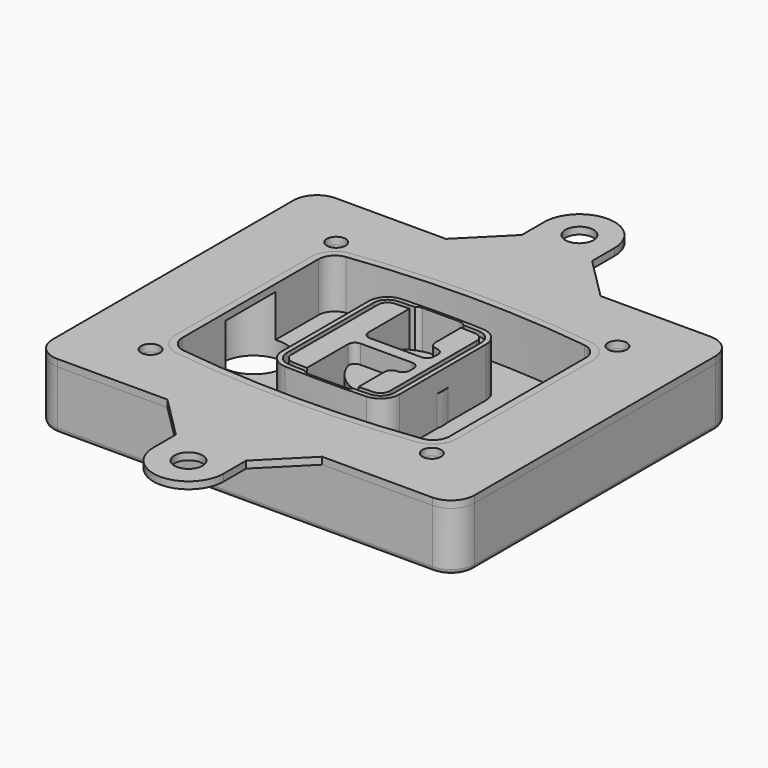
from build123d import *

# Parameters (mm, degrees)
F1_DEPTH  = 25
F2_DEPTH  = 3
F3_DEPTH  = 18
F5_DEPTH  = 21
F6_DEPTH  = 2
F8_DEPTH  = 20
F9_DEPTH  = 16
F10_DEPTH = 25
F7_R      = 6
F7_R_2    = 4
F11_DEPTH = 6
F13_DEPTH = 9
F15_R     = 2
F17_R     = 4
F17_R_2   = 6
F18_DEPTH = 3


# Not quite as in the source:
# - a feature of the source that left no trace in its solid (it failed there, or was rolled back) is left out
# - a feature names something its author has since deleted; it is built from what else it names


with BuildPart() as f1:
    # F0 (on Top) → F1 (new body)
    with BuildSketch(Plane.XY):
        with BuildLine():
            ThreePointArc((-90, -64.25), (-87.0710678119, -71.3210678119), (-80, -74.25))
            Line((-80, -74.25), (80, -74.25))
            ThreePointArc((80, -74.25), (87.0710678119, -71.3210678119), (90, -64.25))
            Line((90, -64.25), (90, 64.25))
            ThreePointArc((90, 64.25), (87.0710678119, 71.3210678119), (80, 74.25))
            Line((80, 74.25), (-80, 74.25))
            ThreePointArc((-80, 74.25), (-87.0710678119, 71.3210678119), (-90, 64.25))
            Line((-90, 64.25), (-90, -64.25))
        make_face()
        with BuildLine():
            ThreePointArc((-60.5228833457, 45.5343231338), (-62.6370880358, 52.5076181093), (-56, 49.5))
            ThreePointArc((-56, 49.5), (-56.010223193, 49.2142010667), (-56.0408405151, 48.9298630223))
            ThreePointArc((-56.0408405151, 48.9298630223), (-53.9627965672, 49.7276492937), (-51.7845761632, 50.1860000938))
            ThreePointArc((-51.7845761632, 50.1860000938), (0, 53.5), (51.7845761632, 50.1860000938))
            ThreePointArc((51.7845761632, 50.1860000938), (53.9627965672, 49.7276492937), (56.0408405151, 48.9298630223))
            ThreePointArc((56.0408405151, 48.9298630223), (59.7142010667, 53.489776807), (64, 49.5))
            ThreePointArc((64, 49.5), (63.0076181093, 46.8629119642), (60.5228833457, 45.5343231338))
            ThreePointArc((60.5228833457, 45.5343231338), (63.1019152577, 41.2337455934), (64, 36.300205629))
            Line((64, 36.300205629), (64, -36.300205629))
            ThreePointArc((64, -36.300205629), (63.1019152577, -41.2337455934), (60.5228833457, -45.5343231338))
            ThreePointArc((60.5228833457, -45.5343231338), (63.0076181093, -46.8629119642), (64, -49.5))
            ThreePointArc((64, -49.5), (59.7142010667, -53.489776807), (56.0408405151, -48.9298630223))
            ThreePointArc((56.0408405151, -48.9298630223), (53.9627965672, -49.7276492937), (51.7845761632, -50.1860000938))
            ThreePointArc((51.7845761632, -50.1860000938), (0, -53.5), (-51.7845761632, -50.1860000938))
            ThreePointArc((-51.7845761632, -50.1860000938), (-53.9627965672, -49.7276492937), (-56.0408405151, -48.9298630223))
            ThreePointArc((-56.0408405151, -48.9298630223), (-56.010223193, -49.2142010667), (-56, -49.5))
            ThreePointArc((-56, -49.5), (-62.6370880358, -52.5076181093), (-60.5228833457, -45.5343231338))
            ThreePointArc((-60.5228833457, -45.5343231338), (-63.1019152577, -41.2337455934), (-64, -36.300205629))
            Line((-64, -36.300205629), (-64, 36.300205629))
            ThreePointArc((-64, 36.300205629), (-63.1019152577, 41.2337455934), (-60.5228833457, 45.5343231338))
        make_face(mode=Mode.SUBTRACT)
        with BuildLine():
            ThreePointArc((-56.0408405151, 48.9298630223), (-57.584545341, 46.3116495189), (-60.5228833457, 45.5343231338))
            ThreePointArc((-60.5228833457, 45.5343231338), (-63.1019152577, 41.2337455934), (-64, 36.300205629))
            Line((-64, 36.300205629), (-64, -36.300205629))
            ThreePointArc((-64, -36.300205629), (-63.1019152577, -41.2337455934), (-60.5228833457, -45.5343231338))
            ThreePointArc((-60.5228833457, -45.5343231338), (-57.584545341, -46.3116495189), (-56.0408405151, -48.9298630223))
            ThreePointArc((-56.0408405151, -48.9298630223), (-53.9627965672, -49.7276492937), (-51.7845761632, -50.1860000938))
            ThreePointArc((-51.7845761632, -50.1860000938), (0, -53.5), (51.7845761632, -50.1860000938))
            ThreePointArc((51.7845761632, -50.1860000938), (53.9627965672, -49.7276492937), (56.0408405151, -48.9298630223))
            ThreePointArc((56.0408405151, -48.9298630223), (57.584545341, -46.3116495189), (60.5228833457, -45.5343231338))
            ThreePointArc((60.5228833457, -45.5343231338), (63.1019152577, -41.2337455934), (64, -36.300205629))
            Line((64, -36.300205629), (64, 36.300205629))
            ThreePointArc((64, 36.300205629), (63.1019152577, 41.2337455934), (60.5228833457, 45.5343231338))
            ThreePointArc((60.5228833457, 45.5343231338), (57.584545341, 46.3116495189), (56.0408405151, 48.9298630223))
            ThreePointArc((56.0408405151, 48.9298630223), (53.9627965672, 49.7276492937), (51.7845761632, 50.1860000938))
            ThreePointArc((51.7845761632, 50.1860000938), (0, 53.5), (-51.7845761632, 50.1860000938))
            ThreePointArc((-51.7845761632, 50.1860000938), (-53.9627965672, 49.7276492937), (-56.0408405151, 48.9298630223))
        make_face()
        with BuildLine():
            Line((-60, -36.300205629), (-60, 36.300205629))
            ThreePointArc((-60, 36.300205629), (-57.5082279066, 42.9052426239), (-51.2746972594, 46.2186302467))
            ThreePointArc((-51.2746972594, 46.2186302467), (0, 49.5), (51.2746972594, 46.2186302467))
            ThreePointArc((51.2746972594, 46.2186302467), (57.5082279066, 42.9052426239), (60, 36.300205629))
            Line((60, 36.300205629), (60, -36.300205629))
            ThreePointArc((60, -36.300205629), (57.5082279066, -42.9052426239), (51.2746972594, -46.2186302467))
            ThreePointArc((51.2746972594, -46.2186302467), (0, -49.5), (-51.2746972594, -46.2186302467))
            ThreePointArc((-51.2746972594, -46.2186302467), (-57.5082279066, -42.9052426239), (-60, -36.300205629))
        make_face(mode=Mode.SUBTRACT)
        with BuildLine():
            ThreePointArc((-51.2746972594, 46.2186302467), (-57.5082279066, 42.9052426239), (-60, 36.300205629))
            Line((-60, 36.300205629), (-60, -36.300205629))
            ThreePointArc((-60, -36.300205629), (-57.5082279066, -42.9052426239), (-51.2746972594, -46.2186302467))
            ThreePointArc((-51.2746972594, -46.2186302467), (0, -49.5), (51.2746972594, -46.2186302467))
            ThreePointArc((51.2746972594, -46.2186302467), (57.5082279066, -42.9052426239), (60, -36.300205629))
            Line((60, -36.300205629), (60, 36.300205629))
            ThreePointArc((60, 36.300205629), (57.5082279066, 42.9052426239), (51.2746972594, 46.2186302467))
            ThreePointArc((51.2746972594, 46.2186302467), (0, 49.5), (-51.2746972594, 46.2186302467))
        make_face()
        with BuildLine():
            ThreePointArc((50.8922880816, 43.2431028614), (55.2557595346, 40.9237315254), (57, 36.300205629))
            Line((57, 36.300205629), (57, -36.300205629))
            ThreePointArc((57, -36.300205629), (55.2557595346, -40.9237315254), (50.8922880816, -43.2431028614))
            ThreePointArc((50.8922880816, -43.2431028614), (0, -46.5), (-50.8922880816, -43.2431028614))
            ThreePointArc((-50.8922880816, -43.2431028614), (-55.2557595346, -40.9237315254), (-57, -36.300205629))
            Line((-57, -36.300205629), (-57, 36.300205629))
            ThreePointArc((-57, 36.300205629), (-55.2557595346, 40.9237315254), (-50.8922880816, 43.2431028614))
            ThreePointArc((-50.8922880816, 43.2431028614), (0, 46.5), (50.8922880816, 43.2431028614))
        make_face(mode=Mode.SUBTRACT)
        with BuildLine():
            Line((57, -36.300205629), (57, 36.300205629))
            ThreePointArc((57, 36.300205629), (55.2557595346, 40.9237315254), (50.8922880816, 43.2431028614))
            ThreePointArc((50.8922880816, 43.2431028614), (0, 46.5), (-50.8922880816, 43.2431028614))
            ThreePointArc((-50.8922880816, 43.2431028614), (-55.2557595346, 40.9237315254), (-57, 36.300205629))
            Line((-57, 36.300205629), (-57, -36.300205629))
            ThreePointArc((-57, -36.300205629), (-55.2557595346, -40.9237315254), (-50.8922880816, -43.2431028614))
            ThreePointArc((-50.8922880816, -43.2431028614), (0, -46.5), (50.8922880816, -43.2431028614))
            ThreePointArc((50.8922880816, -43.2431028614), (55.2557595346, -40.9237315254), (57, -36.300205629))
        make_face()
    extrude(amount=-F1_DEPTH)

    # F0 (on Top) → F2 (join)
    with BuildSketch(Plane.XY):
        with BuildLine():
            ThreePointArc((-51.2746972594, 46.2186302467), (-57.5082279066, 42.9052426239), (-60, 36.300205629))
            Line((-60, 36.300205629), (-60, -36.300205629))
            ThreePointArc((-60, -36.300205629), (-57.5082279066, -42.9052426239), (-51.2746972594, -46.2186302467))
            ThreePointArc((-51.2746972594, -46.2186302467), (0, -49.5), (51.2746972594, -46.2186302467))
            ThreePointArc((51.2746972594, -46.2186302467), (57.5082279066, -42.9052426239), (60, -36.300205629))
            Line((60, -36.300205629), (60, 36.300205629))
            ThreePointArc((60, 36.300205629), (57.5082279066, 42.9052426239), (51.2746972594, 46.2186302467))
            ThreePointArc((51.2746972594, 46.2186302467), (0, 49.5), (-51.2746972594, 46.2186302467))
        make_face()
        with BuildLine():
            ThreePointArc((50.8922880816, 43.2431028614), (55.2557595346, 40.9237315254), (57, 36.300205629))
            Line((57, 36.300205629), (57, -36.300205629))
            ThreePointArc((57, -36.300205629), (55.2557595346, -40.9237315254), (50.8922880816, -43.2431028614))
            ThreePointArc((50.8922880816, -43.2431028614), (0, -46.5), (-50.8922880816, -43.2431028614))
            ThreePointArc((-50.8922880816, -43.2431028614), (-55.2557595346, -40.9237315254), (-57, -36.300205629))
            Line((-57, -36.300205629), (-57, 36.300205629))
            ThreePointArc((-57, 36.300205629), (-55.2557595346, 40.9237315254), (-50.8922880816, 43.2431028614))
            ThreePointArc((-50.8922880816, 43.2431028614), (0, 46.5), (50.8922880816, 43.2431028614))
        make_face(mode=Mode.SUBTRACT)
    extrude(amount=F2_DEPTH)

    # F0 (on Top) → F3 (cut)
    with BuildSketch(Plane.XY):
        with BuildLine():
            Line((57, -36.300205629), (57, 36.300205629))
            ThreePointArc((57, 36.300205629), (55.2557595346, 40.9237315254), (50.8922880816, 43.2431028614))
            ThreePointArc((50.8922880816, 43.2431028614), (0, 46.5), (-50.8922880816, 43.2431028614))
            ThreePointArc((-50.8922880816, 43.2431028614), (-55.2557595346, 40.9237315254), (-57, 36.300205629))
            Line((-57, 36.300205629), (-57, -36.300205629))
            ThreePointArc((-57, -36.300205629), (-55.2557595346, -40.9237315254), (-50.8922880816, -43.2431028614))
            ThreePointArc((-50.8922880816, -43.2431028614), (0, -46.5), (50.8922880816, -43.2431028614))
            ThreePointArc((50.8922880816, -43.2431028614), (55.2557595346, -40.9237315254), (57, -36.300205629))
        make_face()
    extrude(amount=-F3_DEPTH, mode=Mode.SUBTRACT)

    # F4 (on face) → F5 (join, through all)
    with BuildSketch(Plane.XY.offset(3)):
        with BuildLine():
            ThreePointArc((-25, -23.1157506345), (-22.7832384679, -28.6433317351), (-17.361461794, -31.1075805483))
            ThreePointArc((-17.361461794, -31.1075805483), (0, -31.5), (17.361461794, -31.1075805483))
            ThreePointArc((17.361461794, -31.1075805483), (22.7832384679, -28.6433317351), (25, -23.1157506345))
            Line((25, -23.1157506345), (25, 23.1157506345))
            ThreePointArc((25, 23.1157506345), (22.7832384679, 28.6433317351), (17.361461794, 31.1075805483))
            ThreePointArc((17.361461794, 31.1075805483), (0, 31.5), (-17.361461794, 31.1075805483))
            ThreePointArc((-17.361461794, 31.1075805483), (-22.7832384679, 28.6433317351), (-25, 23.1157506345))
            Line((-25, 23.1157506345), (-25, -23.1157506345))
        make_face()
        with BuildLine():
            ThreePointArc((17.2710963455, 29.1096230698), (21.3374288509, 27.2614364599), (23, 23.1157506345))
            Line((23, 23.1157506345), (23, -23.1157506345))
            ThreePointArc((23, -23.1157506345), (21.3374288509, -27.2614364599), (17.2710963455, -29.1096230698))
            ThreePointArc((17.2710963455, -29.1096230698), (13.8131178726, -29.2503406735), (10.354007104, -29.3597447552))
            ThreePointArc((10.354007104, -29.3597447552), (9.3078160678, -30.1999290977), (8, -30.5))
            Line((8, -30.5), (-8, -30.5))
            ThreePointArc((-8, -30.5), (-9.3078160678, -30.1999290977), (-10.354007104, -29.3597447552))
            ThreePointArc((-10.354007104, -29.3597447552), (-13.8131178726, -29.2503406735), (-17.2710963455, -29.1096230698))
            ThreePointArc((-17.2710963455, -29.1096230698), (-21.3374288509, -27.2614364599), (-23, -23.1157506345))
            Line((-23, -23.1157506345), (-23, 23.1157506345))
            ThreePointArc((-23, 23.1157506345), (-21.3374288509, 27.2614364599), (-17.2710963455, 29.1096230698))
            ThreePointArc((-17.2710963455, 29.1096230698), (-13.8131178726, 29.2503406735), (-10.354007104, 29.3597447552))
            ThreePointArc((-10.354007104, 29.3597447552), (-9.3078160678, 30.1999290977), (-8, 30.5))
            Line((-8, 30.5), (8, 30.5))
            ThreePointArc((8, 30.5), (9.3078160678, 30.1999290977), (10.354007104, 29.3597447552))
            ThreePointArc((10.354007104, 29.3597447552), (13.8131178726, 29.2503406735), (17.2710963455, 29.1096230698))
        make_face(mode=Mode.SUBTRACT)
        with BuildLine():
            Line((23, -23.1157506345), (23, 23.1157506345))
            ThreePointArc((23, 23.1157506345), (21.3374288509, 27.2614364599), (17.2710963455, 29.1096230698))
            ThreePointArc((17.2710963455, 29.1096230698), (13.8131178726, 29.2503406735), (10.354007104, 29.3597447552))
            ThreePointArc((10.354007104, 29.3597447552), (10.8339037838, 28.4843725637), (11, 27.5))
            Line((11, 27.5), (11, 27.3408608478))
            ThreePointArc((11, 27.3408608478), (14.0908314548, 27.2388300581), (17.180730897, 27.1116655914))
            ThreePointArc((17.180730897, 27.1116655914), (19.8916192339, 25.8795411848), (21, 23.1157506345))
            Line((21, 23.1157506345), (21, -23.1157506345))
            ThreePointArc((21, -23.1157506345), (19.8916192339, -25.8795411848), (17.180730897, -27.1116655914))
            ThreePointArc((17.180730897, -27.1116655914), (14.0908314548, -27.2388300581), (11, -27.3408608478))
            Line((11, -27.3408608478), (11, -27.5))
            ThreePointArc((11, -27.5), (10.8339037838, -28.4843725637), (10.354007104, -29.3597447552))
            ThreePointArc((10.354007104, -29.3597447552), (13.8131178726, -29.2503406735), (17.2710963455, -29.1096230698))
            ThreePointArc((17.2710963455, -29.1096230698), (21.3374288509, -27.2614364599), (23, -23.1157506345))
        make_face()
        with BuildLine():
            ThreePointArc((17.180730897, 27.1116655914), (14.0908314548, 27.2388300581), (11, 27.3408608478))
            Line((11, 27.3408608478), (11, 13.5))
            ThreePointArc((11, 13.5), (11.8786796564, 11.3786796564), (14, 10.5))
            ThreePointArc((14, 10.5), (16.1213203436, 9.6213203436), (17, 7.5))
            Line((17, 7.5), (17, 5.5))
            ThreePointArc((17, 5.5), (16.1213203436, 3.3786796564), (14, 2.5))
            Line((14, 2.5), (-8, 2.5))
            ThreePointArc((-8, 2.5), (-10.1213203436, 3.3786796564), (-11, 5.5))
            Line((-11, 5.5), (-11, 27.3408608478))
            ThreePointArc((-11, 27.3408608478), (-14.0908314548, 27.2388300581), (-17.180730897, 27.1116655914))
            ThreePointArc((-17.180730897, 27.1116655914), (-19.8916192339, 25.8795411848), (-21, 23.1157506345))
            Line((-21, 23.1157506345), (-21, -23.1157506345))
            ThreePointArc((-21, -23.1157506345), (-19.8916192339, -25.8795411848), (-17.180730897, -27.1116655914))
            ThreePointArc((-17.180730897, -27.1116655914), (-14.0908314548, -27.2388300581), (-11, -27.3408608478))
            Line((-11, -27.3408608478), (-11, -5.5))
            ThreePointArc((-11, -5.5), (-10.1213203436, -3.3786796564), (-8, -2.5))
            Line((-8, -2.5), (14, -2.5))
            ThreePointArc((14, -2.5), (16.1213203436, -3.3786796564), (17, -5.5))
            Line((17, -5.5), (17, -7.5))
            ThreePointArc((17, -7.5), (16.1213203436, -9.6213203436), (14, -10.5))
            ThreePointArc((14, -10.5), (11.8786796564, -11.3786796564), (11, -13.5))
            Line((11, -13.5), (11, -27.3408608478))
            ThreePointArc((11, -27.3408608478), (14.0908314548, -27.2388300581), (17.180730897, -27.1116655914))
            ThreePointArc((17.180730897, -27.1116655914), (19.8916192339, -25.8795411848), (21, -23.1157506345))
            Line((21, -23.1157506345), (21, 23.1157506345))
            ThreePointArc((21, 23.1157506345), (19.8916192339, 25.8795411848), (17.180730897, 27.1116655914))
        make_face()
    extrude(amount=-F5_DEPTH)

    # F4 (on face) → F6 (cut)
    with BuildSketch(Plane.XY.offset(3)):
        with BuildLine():
            Line((23, -23.1157506345), (23, 23.1157506345))
            ThreePointArc((23, 23.1157506345), (21.3374288509, 27.2614364599), (17.2710963455, 29.1096230698))
            ThreePointArc((17.2710963455, 29.1096230698), (13.8131178726, 29.2503406735), (10.354007104, 29.3597447552))
            ThreePointArc((10.354007104, 29.3597447552), (10.8339037838, 28.4843725637), (11, 27.5))
            Line((11, 27.5), (11, 27.3408608478))
            ThreePointArc((11, 27.3408608478), (14.0908314548, 27.2388300581), (17.180730897, 27.1116655914))
            ThreePointArc((17.180730897, 27.1116655914), (19.8916192339, 25.8795411848), (21, 23.1157506345))
            Line((21, 23.1157506345), (21, -23.1157506345))
            ThreePointArc((21, -23.1157506345), (19.8916192339, -25.8795411848), (17.180730897, -27.1116655914))
            ThreePointArc((17.180730897, -27.1116655914), (14.0908314548, -27.2388300581), (11, -27.3408608478))
            Line((11, -27.3408608478), (11, -27.5))
            ThreePointArc((11, -27.5), (10.8339037838, -28.4843725637), (10.354007104, -29.3597447552))
            ThreePointArc((10.354007104, -29.3597447552), (13.8131178726, -29.2503406735), (17.2710963455, -29.1096230698))
            ThreePointArc((17.2710963455, -29.1096230698), (21.3374288509, -27.2614364599), (23, -23.1157506345))
        make_face()
    extrude(amount=-F6_DEPTH, mode=Mode.SUBTRACT)

    # F7 (on face) → F8 (join)
    with BuildSketch(Plane(origin=(0, 0, -25), x_dir=(1, 0, 0), z_dir=(0, 0, -1))):
        with BuildLine():
            ThreePointArc((-6.71157564, 0), (6.7567035675, 13.4682792075), (20.224982775, 0))
            Line((20.224982775, 0), (25.224982775, 0))
            ThreePointArc((25.224982775, 0), (6.7567035675, 18.4682792075), (-11.71157564, 0))
            Line((-11.71157564, 0), (-6.71157564, 0))
        make_face()
        with BuildLine():
            Line((-6.71157564, 0), (20.224982775, 0))
            ThreePointArc((20.224982775, 0), (6.7567035675, 13.4682792075), (-6.71157564, 0))
        make_face()
        with BuildLine():
            ThreePointArc((-6.71157564, 0), (6.7567035675, -13.4682792075), (20.224982775, 0))
            Line((20.224982775, 0), (-6.71157564, 0))
        make_face()
        with BuildLine():
            Line((25.224982775, 0), (20.224982775, 0))
            ThreePointArc((20.224982775, 0), (6.7567035675, -13.4682792075), (-6.71157564, 0))
            Line((-6.71157564, 0), (-11.71157564, 0))
            ThreePointArc((-11.71157564, 0), (6.7567035675, -18.4682792075), (25.224982775, 0))
        make_face()
    extrude(amount=-F8_DEPTH)

    # F7 (on face) → F9 (cut)
    with BuildSketch(Plane(origin=(0, 0, -25), x_dir=(1, 0, 0), z_dir=(0, 0, -1))):
        with BuildLine():
            Line((-6.71157564, 0), (20.224982775, 0))
            ThreePointArc((20.224982775, 0), (6.7567035675, 13.4682792075), (-6.71157564, 0))
        make_face()
        with BuildLine():
            ThreePointArc((-6.71157564, 0), (6.7567035675, -13.4682792075), (20.224982775, 0))
            Line((20.224982775, 0), (-6.71157564, 0))
        make_face()
    extrude(amount=-F9_DEPTH, mode=Mode.SUBTRACT)

    # F7 (on face) → F10 (cut)
    with BuildSketch(Plane(origin=(0, 0, -25), x_dir=(1, 0, 0), z_dir=(0, 0, -1))):
        with BuildLine():
            Line((-69.0318229325, 0), (-42.0952645175, 0))
            ThreePointArc((-42.0952645175, 0), (-55.563543725, 13.4682792075), (-69.0318229325, 0))
        make_face()
        with BuildLine():
            ThreePointArc((-69.0318229325, 0), (-55.563543725, -13.4682792075), (-42.0952645175, 0))
            Line((-42.0952645175, 0), (-69.0318229325, 0))
        make_face()
    extrude(amount=-F10_DEPTH, mode=Mode.SUBTRACT)

    # F7 (on face) → F11 (cut)
    with BuildSketch(Plane(origin=(0, 0, -25), x_dir=(1, 0, 0), z_dir=(0, 0, -1))):
        with Locations((60, -49.5)):
            Circle(F7_R)
        with Locations((60, -49.5)):
            Circle(F7_R_2, mode=Mode.SUBTRACT)
        with Locations((-60, -49.5)):
            Circle(F7_R)
        with Locations((-60, -49.5)):
            Circle(F7_R_2, mode=Mode.SUBTRACT)
        with Locations((-60, 49.5)):
            Circle(F7_R)
        with Locations((-60, 49.5)):
            Circle(F7_R_2, mode=Mode.SUBTRACT)
        with Locations((60, 49.5)):
            Circle(F7_R)
        with Locations((60, 49.5)):
            Circle(F7_R_2, mode=Mode.SUBTRACT)
    extrude(amount=-F11_DEPTH, mode=Mode.SUBTRACT)

    # F12 (on face) → F13 (cut, through all)
    with BuildSketch(Plane(origin=(0, 0, -9), x_dir=(1, 0, 0), z_dir=(0, 0, -1))):
        with BuildLine():
            ThreePointArc((20.224982775, 0), (20.1663399806, 1.2554664788), (19.9909222755, 2.5))
            Line((19.9909222755, 2.5), (14, 2.5))
            ThreePointArc((14, 2.5), (16.1213203436, 3.3786796564), (17, 5.5))
            Line((17, 5.5), (17, 7.5))
            ThreePointArc((17, 7.5), (16.1213203436, 9.6213203436), (14, 10.5))
            ThreePointArc((14, 10.5), (12.1627255951, 11.1284134507), (11.0951631559, 12.750384826))
            ThreePointArc((11.0951631559, 12.750384826), (11.0476113807, 12.7664660322), (11, 12.7823698976))
            Line((11, 12.7823698976), (11, -12.7823698976))
            ThreePointArc((11, -12.7823698976), (11.0476113807, -12.7664660322), (11.0951631559, -12.750384826))
            ThreePointArc((11.0951631559, -12.750384826), (12.1627255951, -11.1284134507), (14, -10.5))
            ThreePointArc((14, -10.5), (16.1213203436, -9.6213203436), (17, -7.5))
            Line((17, -7.5), (17, -5.5))
            ThreePointArc((17, -5.5), (16.1213203436, -3.3786796564), (14, -2.5))
            Line((14, -2.5), (19.9909222755, -2.5))
            ThreePointArc((19.9909222755, -2.5), (20.1663399806, -1.2554664788), (20.224982775, 0))
        make_face()
    extrude(amount=F13_DEPTH, mode=Mode.SUBTRACT)

    # F15
    f15_edges = [f1.edges().sort_by_distance(p)[0] for p in [
        (0, -74.25, -25),
        (-87.071068, -71.321068, -25),
        (-90, 0, -25),
        (-87.071068, 71.321068, -25),
        (87.071068, -71.321068, -25),
        (0, 74.25, -25),
        (90, 0, -25),
        (87.071068, 71.321068, -25),
    ]]
    fillet(f15_edges, radius=F15_R)


with BuildPart() as f18:
    # F17 (on face) → F18 (new body, through all)
    with BuildSketch(Plane.XY):
        with BuildLine():
            Line((-33, 74.25), (-80, 74.25))
            ThreePointArc((-80, 74.25), (-87.0710678119, 71.3210678119), (-90, 64.25))
            Line((-90, 64.25), (-90, -64.25))
            ThreePointArc((-90, -64.25), (-87.0710678119, -71.3210678119), (-80, -74.25))
            Line((-80, -74.25), (-33, -74.25))
            Line((-33, -74.25), (33, -74.25))
            Line((33, -74.25), (80, -74.25))
            ThreePointArc((80, -74.25), (87.0710678119, -71.3210678119), (90, -64.25))
            Line((90, -64.25), (90, 64.25))
            ThreePointArc((90, 64.25), (87.0710678119, 71.3210678119), (80, 74.25))
            Line((80, 74.25), (33, 74.25))
            Line((33, 74.25), (-33, 74.25))
        make_face()
        with Locations((-60, -49.5)):
            Circle(F17_R, mode=Mode.SUBTRACT)
        with Locations((60, -49.5)):
            Circle(F17_R, mode=Mode.SUBTRACT)
        with Locations((-60, 49.5)):
            Circle(F17_R, mode=Mode.SUBTRACT)
        with BuildLine():
            Line((-60, -36.300205629), (-60, 36.300205629))
            ThreePointArc((-60, 36.300205629), (-57.5082279066, 42.9052426239), (-51.2746972594, 46.2186302467))
            ThreePointArc((-51.2746972594, 46.2186302467), (0, 49.5), (51.2746972594, 46.2186302467))
            ThreePointArc((51.2746972594, 46.2186302467), (57.5082279066, 42.9052426239), (60, 36.300205629))
            Line((60, 36.300205629), (60, -36.300205629))
            ThreePointArc((60, -36.300205629), (57.5082279066, -42.9052426239), (51.2746972594, -46.2186302467))
            ThreePointArc((51.2746972594, -46.2186302467), (0, -49.5), (-51.2746972594, -46.2186302467))
            ThreePointArc((-51.2746972594, -46.2186302467), (-57.5082279066, -42.9052426239), (-60, -36.300205629))
        make_face(mode=Mode.SUBTRACT)
        with Locations((60, 49.5)):
            Circle(F17_R, mode=Mode.SUBTRACT)
        with BuildLine():
            Line((-15, 92.25), (-33, 74.25))
            Line((-33, 74.25), (33, 74.25))
            Line((33, 74.25), (15, 92.25))
            Line((15, 92.25), (15, 104.25))
            ThreePointArc((15, 104.25), (0, 119.25), (-15, 104.25))
            Line((-15, 104.25), (-15, 92.25))
        make_face()
        with Locations((0, 104.25)):
            Circle(F17_R_2, mode=Mode.SUBTRACT)
        with BuildLine():
            Line((33, -74.25), (-33, -74.25))
            Line((-33, -74.25), (-15, -92.25))
            Line((-15, -92.25), (-15, -104.25))
            ThreePointArc((-15, -104.25), (0, -119.25), (15, -104.25))
            Line((15, -104.25), (15, -92.25))
            Line((15, -92.25), (33, -74.25))
        make_face()
        with Locations((0, -104.25)):
            Circle(F17_R_2, mode=Mode.SUBTRACT)
    extrude(amount=F18_DEPTH)


solid = Compound([f1.part, f18.part])
